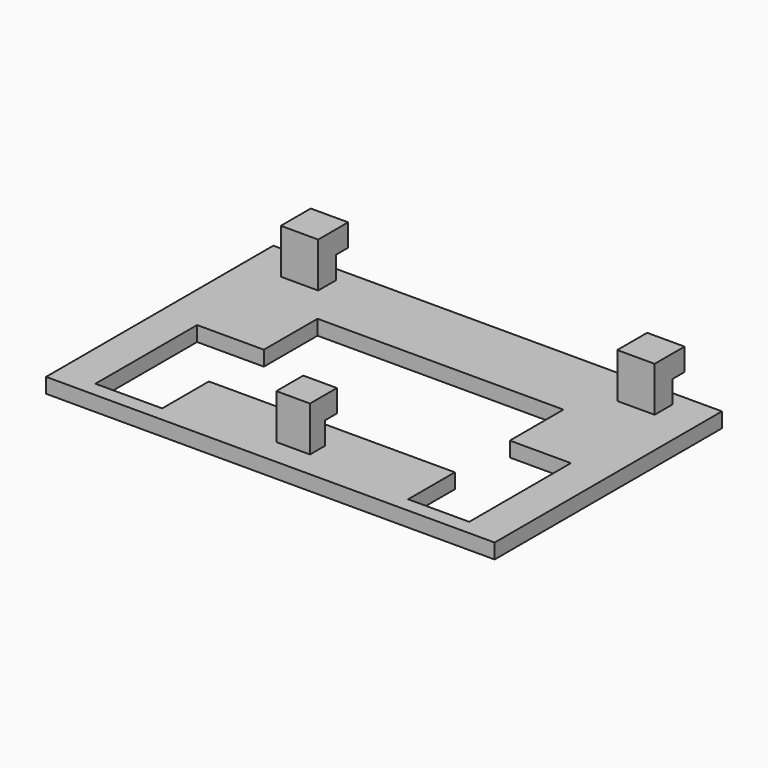
from build123d import *

# Parameters (mm, degrees)
F0_W     = 60
F0_H     = 38
F0_W_2   = 4.5
F0_H_2   = 2.5
F0_W_3   = 5
F0_H_3   = 3
F1_DEPTH = 2
F2_DEPTH = 8
F3_W     = 5
F3_H     = 3
F4_DEPTH = 2
F5_W     = 5
F5_H     = 3
F6_DEPTH = 2
F7_DEPTH = 8
F8_W     = 4.5
F8_H     = 3
F9_DEPTH = 2


# Not quite as in the source:
# - a feature names something its author has since deleted; it is built from what else it names


with BuildPart() as f1:
    # F0 (on Top) → F1 (new body)
    with BuildSketch(Plane.XY):
        Rectangle(F0_W, F0_H)
        with Locations((0.25, -14.25)):
            Rectangle(F0_W_2, F0_H_2, mode=Mode.SUBTRACT)
        Polygon((-16.0694369525, 0), (-16.0694369525, 8.9702934623), (16.8300806135, 8.9702934623), (16.8300806135, 0), (25, 0), (25, -17), (16.8300806135, -17), (16.8300806135, -9.1921526343), (-16.0694369525, -9.1921526343), (-16.0694369525, -17), (-25, -17), (-25, 0), align=None, mode=Mode.SUBTRACT)
        with Locations((-22.5, 15.5)):
            Rectangle(F0_W_3, F0_H_3, mode=Mode.SUBTRACT)
        with Locations((22.5, 15.5)):
            Rectangle(F0_W_3, F0_H_3, mode=Mode.SUBTRACT)
    extrude(amount=F1_DEPTH)

    # F0 (on Top) → F2 (join)
    with BuildSketch(Plane.XY):
        with Locations((22.5, 15.5)):
            Rectangle(F0_W_3, F0_H_3)
        with Locations((-22.5, 15.5)):
            Rectangle(F0_W_3, F0_H_3)
    extrude(amount=F2_DEPTH)

    # F3 (on face) → F4 (join)
    with BuildSketch(Plane(origin=(0, 17, 0), x_dir=(-1, 0, 0), z_dir=(0, 1, 0))):
        with Locations((22.5, 6.5)):
            Rectangle(F3_W, F3_H)
    extrude(amount=F4_DEPTH)

    # F5 (on face) → F6 (join)
    with BuildSketch(Plane(origin=(0, 17, 0), x_dir=(-1, 0, 0), z_dir=(0, 1, 0))):
        with Locations((-22.5, 6.5)):
            Rectangle(F5_W, F5_H)
    extrude(amount=F6_DEPTH)

    # F0 (on Top) → F7 (join)
    with BuildSketch(Plane.XY):
        with Locations((0.25, -14.25)):
            Rectangle(F0_W_2, F0_H_2)
    extrude(amount=F7_DEPTH)

    # F8 (on face) → F9 (join)
    with BuildSketch(Plane(origin=(0, -13, 0), x_dir=(-1, 0, 0), z_dir=(0, 1, 0))):
        with Locations((-0.25, 6.5)):
            Rectangle(F8_W, F8_H)
    extrude(amount=F9_DEPTH)


solid = f1.part
